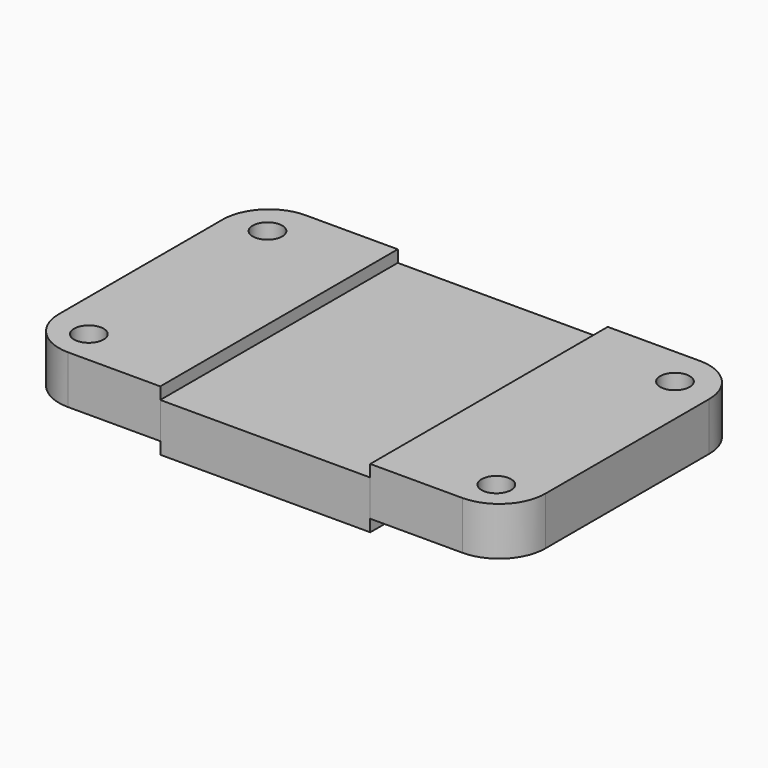
from build123d import *

# Parameters (mm, degrees)
F0_W     = 38.1
F0_H     = 81.86
F0_R     = 4.0695268365
F1_DEPTH = 13.3
F0_W_2   = 28.95
F2_DEPTH = 10
F3_W     = 57.9
F3_H     = 81.86
F4_DEPTH = 3.3
F5_R     = 12.7
F5_2_R   = 12.7


with BuildPart() as f1:
    # F0 (on Top) → F1 (new body)
    with BuildSketch(Plane.XY):
        with Locations((-48, 0)):
            Rectangle(F0_W, F0_H)
        with Locations((-56.1804731635, -31.5004731635)):
            Circle(F0_R, mode=Mode.SUBTRACT)
        with Locations((-56.1804731635, 30.0604731635)):
            Circle(F0_R, mode=Mode.SUBTRACT)
    extrude(amount=F1_DEPTH)

    # F5
    f5_edges = [f1.edges().sort_by_distance(p)[0] for p in [
        (-67.05, 40.93, 6.65),
        (-67.05, -40.93, 6.65),
    ]]
    fillet(f5_edges, radius=F5_R)


with BuildPart() as f1b:
    # F0 (on Top) → F1, piece 2 (new body)
    with BuildSketch(Plane.XY):
        with Locations((48, 0)):
            Rectangle(F0_W, F0_H)
        with Locations((56.1804731635, -31.5004731635)):
            Circle(F0_R, mode=Mode.SUBTRACT)
        with Locations((56.1804731635, 30.0604731635)):
            Circle(F0_R, mode=Mode.SUBTRACT)
    extrude(amount=F1_DEPTH)

    # F5#2
    f5_2_edges = [f1b.edges().sort_by_distance(p)[0] for p in [
        (67.05, -40.93, 6.65),
        (67.05, 40.93, 6.65),
    ]]
    fillet(f5_2_edges, radius=F5_2_R)


with BuildPart() as f2:
    # F0 (on Top) → F2 (new body)
    with BuildSketch(Plane.XY):
        with Locations((14.475, 0)):
            Rectangle(F0_W_2, F0_H)
        with Locations((-14.475, 0)):
            Rectangle(F0_W_2, F0_H)
    extrude(amount=F2_DEPTH)

    # F3 (on face) → F4 (join)
    with BuildSketch(Plane(origin=(0, 0, 0), x_dir=(1, 0, 0), z_dir=(0, 0, -1))):
        Rectangle(F3_W, F3_H)
    extrude(amount=F4_DEPTH)


solid = Compound([f1.part, f1b.part, f2.part])
